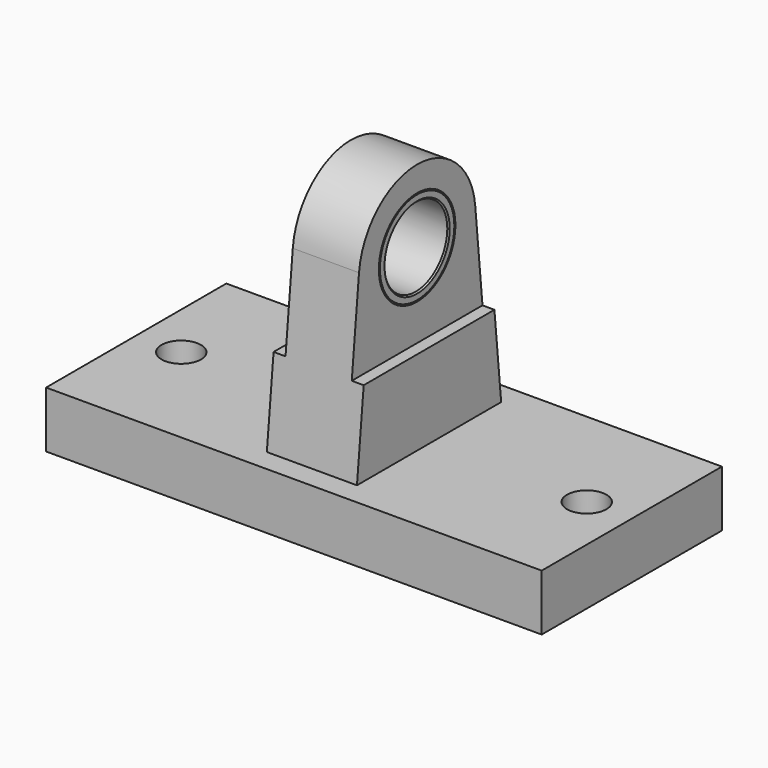
from build123d import *

# Parameters (mm, degrees)
F0_W     = 279.4
F0_H     = 127
F0_R     = 11.1125
F1_DEPTH = 31.75
F2_R     = 26.9875
F3_DEPTH = 18.669
F5_DEPTH = 25.4
F6_R     = 26.9875
F6_R_2   = 22.225
F7_DEPTH = 18.669
F8_SIZE  = 0.762


with BuildPart() as f1:
    # F0 (on Top) → F1 (new body)
    with BuildSketch(Plane.XY):
        Rectangle(F0_W, F0_H)
        with Locations((-114.3, 0)):
            Circle(F0_R, mode=Mode.SUBTRACT)
        with Locations((114.3, 0)):
            Circle(F0_R, mode=Mode.SUBTRACT)
    extrude(amount=-F1_DEPTH)

    # F2 (on Right) → F3 (join, symmetric)
    with BuildSketch(Plane.YZ):
        with BuildLine():
            Line((50.8, 0), (40.9469707894, 99.312448421))
            ThreePointArc((40.9469707894, 99.312448421), (0, 136.398), (-40.9469707894, 99.312448421))
            Line((-40.9469707894, 99.312448421), (-50.8, 0))
            Line((-50.8, 0), (50.8, 0))
        make_face()
        with Locations((0, 95.25)):
            Circle(F2_R, mode=Mode.SUBTRACT)
    extrude(amount=F3_DEPTH, both=True)

    # F4 (on Right) → F5 (join, symmetric)
    with BuildSketch(Plane.YZ):
        Polygon((-50.8, 0), (50.8, 0), (46.0624081035, 47.752), (-46.0624081035, 47.752), align=None)
    extrude(amount=F5_DEPTH, both=True)


with BuildPart() as f7:
    # F6 (on Right) → F7 (new body, symmetric)
    with BuildSketch(Plane.YZ):
        with Locations((0, 95.25)):
            Circle(F6_R)
        with Locations((0, 95.25)):
            Circle(F6_R_2, mode=Mode.SUBTRACT)
    extrude(amount=F7_DEPTH, both=True)

    # F8
    f8_edges = [f7.edges().sort_by_distance(p)[0] for p in [
        (-18.669, -26.9875, 95.25),
        (-18.669, -22.225, 95.25),
        (18.669, -26.9875, 95.25),
        (18.669, -22.225, 95.25),
    ]]
    chamfer(f8_edges, length=F8_SIZE)


solid = Compound([f1.part, f7.part])
